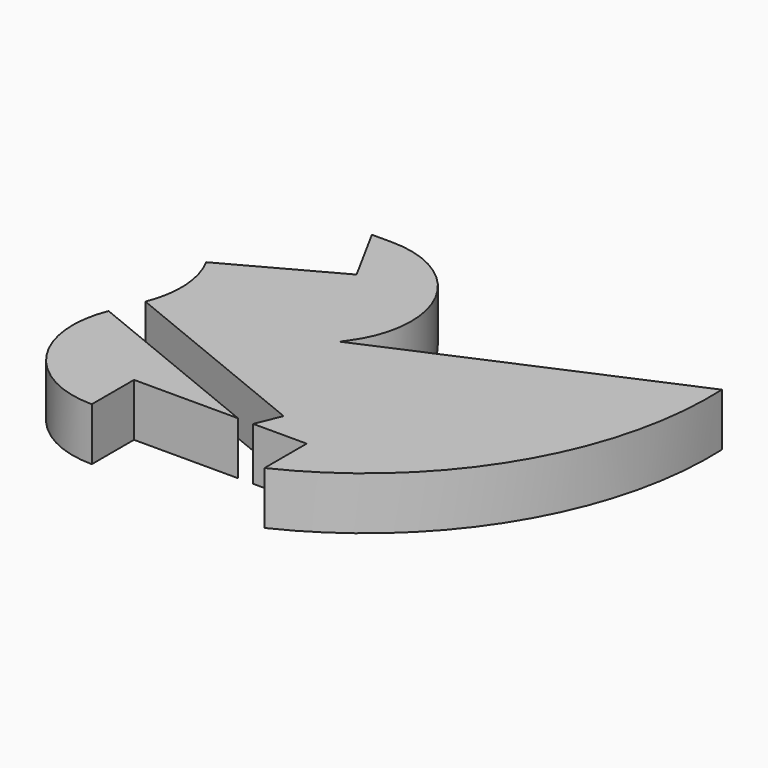
from build123d import *

# Parameters (mm, degrees)
F1_DEPTH    = 25.4
F2_R        = 45.8493910303
F3_DEPTH    = 148.844
F4_DEPTH    = 106.68
F5_DEPTH    = 57.404
F6_T1_DEPTH = 801.4030056795
F7_DEPTH    = 25.4


# Not quite as in the source:
# - a fillet or chamfer that OpenCascade refuses, or shapes differently, is made with other operations: its cross-section is extruded or revolved along the edge and cut away or added


with BuildPart() as f1:
    # F0 (on Top) → F1 (new body)
    with BuildSketch(Plane.XY):
        with BuildLine():
            Line((-75.0448331237, -76.2676075101), (0, 0))
            add(Edge.make_bspline(
                [(0, 0), (-17.1607195909, -0.0678450845), (-34.6268538829, 9.7280369702), (-35.0408777595, 21.7053014785)],
                knots=[0, 0, 0, 0, 0.2466068587, 0.2466068587, 0.2466068587, 0.2466068587], degree=3))
            Line((-35.0408777595, 21.7053014785), (-75.0448331237, -76.2676075101))
        make_face()
        with BuildLine():
            add(Edge.make_bspline(
                [(0, 0), (-17.1607195909, -0.0678450845), (-34.6268538829, 9.7280369702), (-35.0408777595, 21.7053014785)],
                knots=[0, 0, 0, 0, 0.2466068587, 0.2466068587, 0.2466068587, 0.2466068587], degree=3))
            add(Edge.make_bspline(
                [(34.106452018, 21.7053014785), (33.6908138887, 9.8087295701), (16.995182387, 0.0671906315), (0, 0)],
                knots=[0.7557719815, 0.7557719815, 0.7557719815, 0.7557719815, 1, 1, 1, 1], degree=3))
            add(Edge.make_bspline(
                [(0, 48.8035753369), (17.42740955, 48.7254776276), (34.5378985933, 34.0543494732), (34.106452018, 21.7053014785)],
                knots=[0.5022549562, 0.5022549562, 0.5022549562, 0.5022549562, 0.7557719815, 0.7557719815, 0.7557719815, 0.7557719815], degree=3))
            add(Edge.make_bspline(
                [(-35.0408777595, 21.7053014785), (-35.4700808114, 34.1216831702), (-17.5739049114, 48.8823295381), (0, 48.8035753369)],
                knots=[0.2466068587, 0.2466068587, 0.2466068587, 0.2466068587, 0.5022549562, 0.5022549562, 0.5022549562, 0.5022549562], degree=3))
        make_face()
        Polygon((76.5672177076, -76.2676075101), (0, 0), (-75.0448331237, -76.2676075101), align=None)
        with BuildLine():
            add(Edge.make_bspline(
                [(34.106452018, 21.7053014785), (33.6908138887, 9.8087295701), (16.995182387, 0.0671906315), (0, 0)],
                knots=[0.7557719815, 0.7557719815, 0.7557719815, 0.7557719815, 1, 1, 1, 1], degree=3))
            Line((0, 0), (76.5672177076, -76.2676075101))
            Line((76.5672177076, -76.2676075101), (34.106452018, 21.7053014785))
        make_face()
        with BuildLine():
            Line((-76.1296525598, 97.1791520715), (-35.0408777595, 21.7053014785))
            add(Edge.make_bspline(
                [(-35.0408777595, 21.7053014785), (-35.4700808114, 34.1216831702), (-17.5739049114, 48.8823295381), (0, 48.8035753369)],
                knots=[0.2466068587, 0.2466068587, 0.2466068587, 0.2466068587, 0.5022549562, 0.5022549562, 0.5022549562, 0.5022549562], degree=3))
            Line((0, 48.8035753369), (0, 97.1791520715))
            Line((0, 97.1791520715), (-76.1296525598, 97.1791520715))
        make_face()
        with BuildLine():
            add(Edge.make_bspline(
                [(0, 48.8035753369), (17.42740955, 48.7254776276), (34.5378985933, 34.0543494732), (34.106452018, 21.7053014785)],
                knots=[0.5022549562, 0.5022549562, 0.5022549562, 0.5022549562, 0.7557719815, 0.7557719815, 0.7557719815, 0.7557719815], degree=3))
            Line((34.106452018, 21.7053014785), (88.9128223062, 97.1791520715))
            Line((88.9128223062, 97.1791520715), (0, 97.1791520715))
            Line((0, 97.1791520715), (0, 48.8035753369))
        make_face()
    extrude(amount=F1_DEPTH)

    # F2
    f2_edges = [f1.edges().sort_by_distance(p)[0] for p in [
        (88.912822, 97.179152, 12.7),
        (-35.040878, 21.705301, 12.7),
        (-75.044833, -76.267608, 12.7),
    ]]
    fillet(f2_edges, radius=F2_R)

    # F3 (add): a face of the model
    f3_faces = [f1.faces().sort_by_distance(p)[0] for p in [
        (55.3368348628, -27.2811530158, 12.7),
    ]]
    extrude(f3_faces, amount=F3_DEPTH)

    # F4 (cut): a face of the model
    f4_faces = [f1.faces().sort_by_distance(p)[0] for p in [
        (-46.2564858481, -5.7626261429, 12.7),
    ]]
    extrude(f4_faces, amount=-F4_DEPTH, mode=Mode.SUBTRACT)

    # F5 (cut): a face of the model
    f5_faces = [f1.faces().sort_by_distance(p)[0] for p in [
        (-60.7872022152, 68.997396576, 12.7),
    ]]
    extrude(f5_faces, amount=-F5_DEPTH, mode=Mode.SUBTRACT)

    # F6: fillet of radius 166.1799763524 on 1 edges, made by hand

    # F6_s2 → F6_t1 (cut)
    with BuildSketch(Plane.XY.offset(-388.0015028397)):
        with BuildLine():
            ThreePointArc((170.6761321798, 80.8936347588), (145.5192693359, -14.4805618017), (70.7348093872, -78.7953320174))
            Line((70.7348093872, -78.7953320174), (213.1368978695, -17.0792742298))
            Line((213.1368978695, -17.0792742298), (170.6761321798, 80.8936347588))
        make_face()
    extrude(amount=F6_T1_DEPTH, mode=Mode.SUBTRACT)

    # F7 (cut): a face of the model
    f7_faces = [f1.faces().sort_by_distance(p)[0] for p in [
        (34.7430737503, -76.2676075101, 12.7),
    ]]
    extrude(f7_faces, amount=-F7_DEPTH, mode=Mode.SUBTRACT)


solid = f1.part
